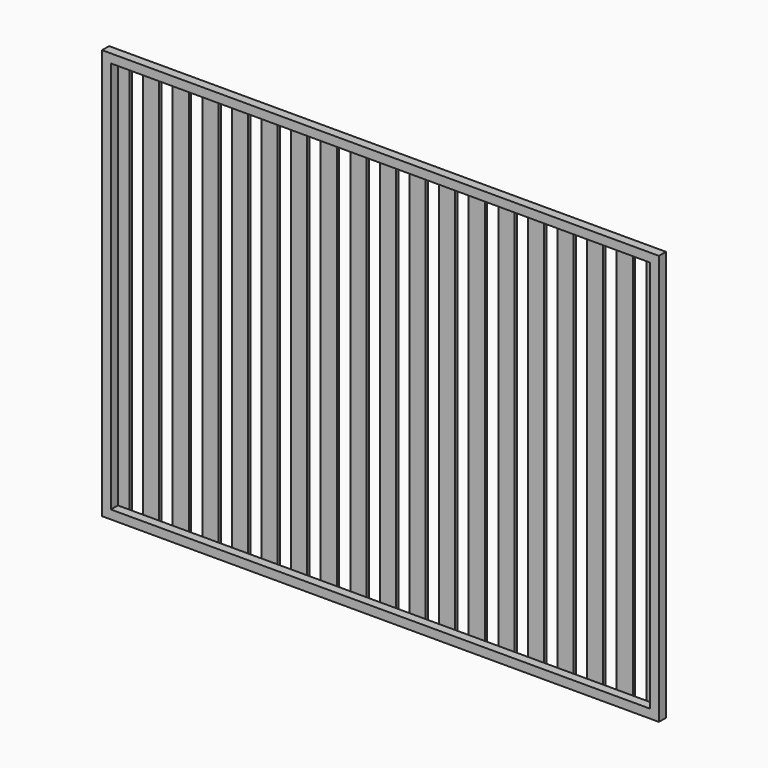
from build123d import *

# Parameters (mm, degrees)
F0_W     = 1900
F0_H     = 1400
F0_W_2   = 1840
F0_H_2   = 1340
F1_DEPTH = 15
F2_W     = 55
F2_H     = 10
F3_DEPTH = 690


# Not quite as in the source:
# - a feature names something its author has since deleted; it is built from what else it names


with BuildPart() as f1:
    # F0 (on Front) → F1 (new body, symmetric)
    with BuildSketch(Plane.XZ):
        Rectangle(F0_W, F0_H)
        Rectangle(F0_W_2, F0_H_2, mode=Mode.SUBTRACT)
    extrude(amount=F1_DEPTH, both=True)

    # F2 (on Top) → F3 (join, symmetric)
    with BuildSketch(Plane.XY):
        with Locations((-907.5, 20)):
            Rectangle(F2_W, F2_H)
        with Locations((-806.5, 20)):
            Rectangle(F2_W, F2_H)
        with Locations((-705.5, 20)):
            Rectangle(F2_W, F2_H)
        with Locations((-604.5, 20)):
            Rectangle(F2_W, F2_H)
        with Locations((-503.5, 20)):
            Rectangle(F2_W, F2_H)
        with Locations((-402.5, 20)):
            Rectangle(F2_W, F2_H)
        with Locations((-301.5, 20)):
            Rectangle(F2_W, F2_H)
        with Locations((-200.5, 20)):
            Rectangle(F2_W, F2_H)
        with Locations((-99.5, 20)):
            Rectangle(F2_W, F2_H)
        with Locations((1.5, 20)):
            Rectangle(F2_W, F2_H)
        with Locations((102.5, 20)):
            Rectangle(F2_W, F2_H)
        with Locations((203.5, 20)):
            Rectangle(F2_W, F2_H)
        with Locations((304.5, 20)):
            Rectangle(F2_W, F2_H)
        with Locations((405.5, 20)):
            Rectangle(F2_W, F2_H)
        with Locations((506.5, 20)):
            Rectangle(F2_W, F2_H)
        with Locations((607.5, 20)):
            Rectangle(F2_W, F2_H)
        with Locations((708.5, 20)):
            Rectangle(F2_W, F2_H)
        with Locations((809.5, 20)):
            Rectangle(F2_W, F2_H)
        with Locations((910.5, 20)):
            Rectangle(F2_W, F2_H)
    extrude(amount=F3_DEPTH, both=True)


solid = f1.part
